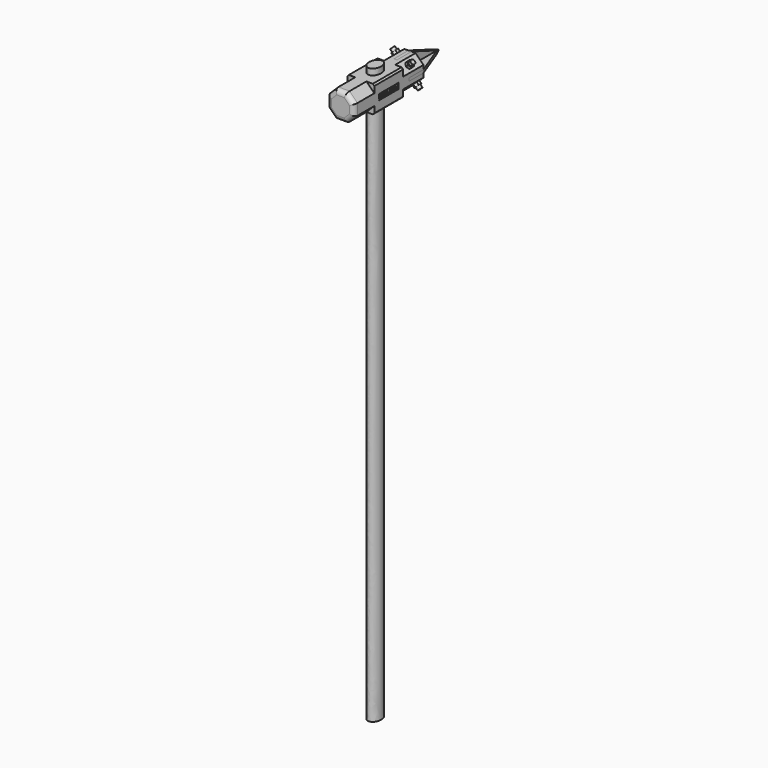
from build123d import *

# Parameters (mm, degrees)
F1_DEPTH       = 1219.2
F3_DEPTH       = 38.1
F3_DEPTH_BACK  = 38.1
F4_DEPTH       = 92.075
F4_DEPTH_BACK  = 92.075
F5_R           = 9.525
F6_SIZE        = 3.175
F7_DEPTH       = 1219.2
F8_W           = 51.7479172142
F8_H           = 12.878934881
F8_W_2         = 48.5729172142
F8_H_2         = 9.703934881
F8_TEXT_SIZE   = 9.0679651125
F9_DEPTH       = 0.79375
F10_W          = 51.7478878901
F10_H          = 12.8789306638
F10_W_2        = 48.5728878901
F10_H_2        = 9.7039306638
F10_TEXT_SIZE  = 9.0679592552
F11_DEPTH      = 0.79375
F13_DEPTH      = 38.1
F14_DEPTH      = 38.1
F15_DEPTH      = 76.2
F17_DEPTH      = 31.75
F17_DEPTH_BACK = 25.4
F19_DEPTH      = 25.4
F20_R          = 4.7625
F21_DEPTH      = 12.7
F21_DEPTH_BACK = 69.85
F22_DEPTH      = 6.35
F23_R          = 4.7625
F24_DEPTH      = 12.7
F24_DEPTH_BACK = 69.85
F25_DEPTH      = 6.35
F26_START      = -63.5
F22_FACE_R     = 4.7625
F26_DEPTH      = 6.35
F27_START      = -63.5
F25_FACE_R     = 4.7625
F27_DEPTH      = 6.35


# Not quite as in the source:
# - Text() gives the source's letters only with a copy of the font that has no kerning and outlines rounded to 1/6400 em; it was checked with that copy


with BuildPart() as f1:
    # F0 (on Top) → F1 (new body)
    with BuildSketch(Plane.XY):
        with BuildLine():
            add(Edge.make_bspline(
                [(12.7, 0), (12.7, 30.2459372272), (-6.35, 15.1229686136), (-25.4, 0), (-6.35, -15.1229686136), (12.7, -30.2459372272), (12.7, 0)],
                knots=[4.7123889804, 4.7123889804, 4.7123889804, 6.8067840828, 6.8067840828, 8.9011791852, 8.9011791852, 10.9955742876, 10.9955742876, 10.9955742876], degree=2, weights=[1, 0.5, 1, 0.5, 1, 0.5, 1]))
        make_face()
    extrude(amount=F1_DEPTH)


with BuildPart() as f3:
    # F2 (on Front) → F3 (new body, two sides)
    with BuildSketch(Plane.XZ) as f3_sk:
        Polygon((-28.575, 1189.7030929186), (-11.8361525448, 1206.4419403738), (-28.575, 1206.4419403738), align=None)
        Polygon((11.8361525448, 1206.4419403738), (28.575, 1189.7030929186), (28.575, 1206.4419403738), align=None)
        Polygon((28.575, 1166.030787829), (28.575, 1189.7030929186), (11.8361525448, 1206.4419403738), (-11.8361525448, 1206.4419403738), (-28.575, 1189.7030929186), (-28.575, 1166.030787829), (-11.8361525448, 1149.2919403738), (11.8361525448, 1149.2919403738), align=None)
        Polygon((-28.575, 1149.2919403738), (-11.8361525448, 1149.2919403738), (-28.575, 1166.030787829), align=None)
        Polygon((28.575, 1149.2919403738), (28.575, 1166.030787829), (11.8361525448, 1149.2919403738), align=None)
    extrude(amount=F3_DEPTH)
    extrude(f3_sk.sketch, amount=-F3_DEPTH_BACK)

    # F2 (on Front) → F4 (join, two sides)
    with BuildSketch(Plane.XZ) as f4_sk:
        Polygon((28.575, 1166.030787829), (28.575, 1189.7030929186), (11.8361525448, 1206.4419403738), (-11.8361525448, 1206.4419403738), (-28.575, 1189.7030929186), (-28.575, 1166.030787829), (-11.8361525448, 1149.2919403738), (11.8361525448, 1149.2919403738), align=None)
    extrude(amount=F4_DEPTH)
    extrude(f4_sk.sketch, amount=-F4_DEPTH_BACK)

    # F5
    f5_edges = [f3.edges().sort_by_distance(p)[0] for p in [
        (20.205576, -92.075, 1157.661364),
        (28.575, -92.075, 1177.86694),
        (20.205576, -92.075, 1198.072517),
        (0, -92.075, 1206.44194),
        (-20.205576, -92.075, 1198.072517),
        (-28.575, -92.075, 1177.86694),
        (-20.205576, -92.075, 1157.661364),
        (0, -92.075, 1149.29194),
    ]]
    fillet(f5_edges, radius=F5_R)

    # F6
    f6_edges = [f3.edges().sort_by_distance(p)[0] for p in [
        (28.575, 0, 1206.44194),
        (28.575, 0, 1149.29194),
        (-28.575, 0, 1206.44194),
        (-28.575, 0, 1149.29194),
    ]]
    chamfer(f6_edges, length=F6_SIZE)

    # F0 (on Top) → F7 (cut)
    with BuildSketch(Plane.XY):
        with BuildLine():
            add(Edge.make_bspline(
                [(12.7, 0), (12.7, 30.2459372272), (-6.35, 15.1229686136), (-25.4, 0), (-6.35, -15.1229686136), (12.7, -30.2459372272), (12.7, 0)],
                knots=[4.7123889804, 4.7123889804, 4.7123889804, 6.8067840828, 6.8067840828, 8.9011791852, 8.9011791852, 10.9955742876, 10.9955742876, 10.9955742876], degree=2, weights=[1, 0.5, 1, 0.5, 1, 0.5, 1]))
        make_face()
    extrude(amount=F7_DEPTH, mode=Mode.SUBTRACT)

    # F8 (on face) → F9 (cut)
    with BuildSketch(Plane.YZ.offset(28.575)):
        with Locations((0, 1177.8669403738)):
            Rectangle(F8_W, F8_H)
        with Locations((0, 1177.8669403738)):
            Rectangle(F8_W_2, F8_H_2, mode=Mode.SUBTRACT)
        with Locations((-22.6989586071, 1174.6024729333)):
            Text('ARTILLIER', F8_TEXT_SIZE, font='Open Sans', font_style=FontStyle.BOLD, text_align=(TextAlign.LEFT, TextAlign.BOTTOM))
    extrude(amount=-F9_DEPTH, mode=Mode.SUBTRACT)

    # F10 (on face) → F11 (cut)
    with BuildSketch(Plane(origin=(-28.575, 0, 0), x_dir=(0, -1, 0), z_dir=(-1, 0, 0))):
        with Locations((0, 1177.925)):
            Rectangle(F10_W, F10_H)
        with Locations((0, 1177.925)):
            Rectangle(F10_W_2, F10_H_2, mode=Mode.SUBTRACT)
        with Locations((-22.6989439451, 1174.6605346681)):
            Text('ARTILLIER', F10_TEXT_SIZE, font='Open Sans', font_style=FontStyle.BOLD, text_align=(TextAlign.LEFT, TextAlign.BOTTOM))
    extrude(amount=-F11_DEPTH, mode=Mode.SUBTRACT)

    # F12 (on face) → F13 (cut)
    with BuildSketch(Plane(origin=(0, 92.075, 0), x_dir=(-1, 0, 0), z_dir=(0, 1, 0))):
        Polygon((-3.175, 1149.2919403738), (3.175, 1149.2919403738), (3.175, 1174.6919403738), (28.575, 1174.6919403738), (28.575, 1181.0419403738), (3.175, 1181.0419403738), (3.175, 1206.4419403738), (-3.175, 1206.4419403738), (-3.175, 1181.0419403738), (-28.575, 1181.0419403738), (-28.575, 1174.6919403738), (-3.175, 1174.6919403738), align=None)
    extrude(amount=-F13_DEPTH, mode=Mode.SUBTRACT)


with BuildPart() as f14:
    # F12 (on face) → F14 (new body)
    with BuildSketch(Plane(origin=(0, 92.075, 0), x_dir=(-1, 0, 0), z_dir=(0, 1, 0))):
        Polygon((-3.175, 1149.2919403738), (3.175, 1149.2919403738), (3.175, 1174.6919403738), (28.575, 1174.6919403738), (28.575, 1181.0419403738), (3.175, 1181.0419403738), (3.175, 1206.4419403738), (-3.175, 1206.4419403738), (-3.175, 1181.0419403738), (-28.575, 1181.0419403738), (-28.575, 1174.6919403738), (-3.175, 1174.6919403738), align=None)
    extrude(amount=-F14_DEPTH)

    # F15 (add): a face of the model
    f15_faces = [f14.faces().sort_by_distance(p)[0] for p in [
        (0, 92.075, 1177.8669403738),
    ]]
    extrude(f15_faces, amount=F15_DEPTH)

    # F16 (on face) → F17 (cut, two sides)
    with BuildSketch(Plane.YZ.offset(3.175)) as f17_sk:
        Polygon((168.275, 1177.8669403738), (168.275, 1181.0419403738), (159.8083333333, 1181.0419403738), align=None)
        Polygon((168.275, 1149.2919403738), (168.275, 1177.8669403738), (92.075, 1149.2919403738), align=None)
        Polygon((168.275, 1181.0419403738), (168.275, 1206.4419403738), (92.075, 1206.4419403738), (159.8083333333, 1181.0419403738), align=None)
    extrude(amount=-F17_DEPTH, mode=Mode.SUBTRACT)
    extrude(f17_sk.sketch, amount=F17_DEPTH_BACK, mode=Mode.SUBTRACT)

    # F18 (on face) → F19 (cut)
    with BuildSketch(Plane.XY.offset(1181.0419403738)):
        Polygon((28.575, 92.075), (28.575, 159.8083333333), (3.175, 159.8083333333), align=None)
        Polygon((-28.575, 92.075), (0, 168.275), (-28.575, 168.275), align=None)
        Polygon((28.575, 159.8083333333), (28.575, 168.275), (0, 168.275), (3.175, 159.8083333333), align=None)
    extrude(amount=-F19_DEPTH, mode=Mode.SUBTRACT)

    # F20 (on face) → F21 (join, two sides)
    with BuildSketch(Plane(origin=(-609.1390464593, 0, 609.1390464593), x_dir=(0, -1, 0), z_dir=(-0.7071067812, 0, 0.7071067812))) as f21_sk:
        with Locations((-82.55, 832.8777008738)):
            Circle(F20_R)
    extrude(amount=F21_DEPTH)
    extrude(f21_sk.sketch, amount=-F21_DEPTH_BACK)

    # F20 (on face) → F22 (join)
    with BuildSketch(Plane(origin=(-609.1390464593, 0, 609.1390464593), x_dir=(0, -1, 0), z_dir=(-0.7071067812, 0, 0.7071067812))):
        Polygon((-86.121875, 826.6910318955), (-78.978125, 826.6910318955), (-75.40625, 832.8777008738), (-78.978125, 839.0643698521), (-86.121875, 839.0643698521), (-89.69375, 832.8777008738), align=None)
        with Locations((-82.55, 832.8777008738)):
            Circle(F20_R, mode=Mode.SUBTRACT)
    extrude(amount=F22_DEPTH)

    # F23 (on face) → F24 (join, two sides)
    with BuildSketch(Plane(origin=(609.1390464593, 0, 609.1390464593), x_dir=(0.7071067812, 0, -0.7071067812), z_dir=(0.7071067812, 0, 0.7071067812))) as f24_sk:
        with Locations((-832.8777008738, 63.5)):
            Circle(F23_R)
    extrude(amount=F24_DEPTH)
    extrude(f24_sk.sketch, amount=-F24_DEPTH_BACK)

    # F23 (on face) → F25 (join)
    with BuildSketch(Plane(origin=(609.1390464593, 0, 609.1390464593), x_dir=(0.7071067812, 0, -0.7071067812), z_dir=(0.7071067812, 0, 0.7071067812))):
        Polygon((-826.6910318955, 59.928125), (-826.6910318955, 67.071875), (-832.8777008738, 70.64375), (-839.0643698521, 67.071875), (-839.0643698521, 59.928125), (-832.8777008738, 56.35625), align=None)
        with Locations((-832.8777008738, 63.5)):
            Circle(F23_R, mode=Mode.SUBTRACT)
    extrude(amount=F25_DEPTH)

    # F22_face (on face) → F26 (join)
    with BuildSketch(Plane(origin=(-24.6957043329, 82.55, 1202.5626447068), x_dir=(0, -1, 0), z_dir=(-0.7071067812, 0, 0.7071067812)).offset(F26_START)):
        Polygon((-3.571875, -6.1866689783), (3.571875, -6.1866689783), (7.14375, 0), (3.571875, 6.1866689783), (-3.571875, 6.1866689783), (-7.14375, 0), align=None)
        Circle(F22_FACE_R, mode=Mode.SUBTRACT)
    extrude(amount=-F26_DEPTH)

    # F25_face (on face) → F27 (join)
    with BuildSketch(Plane(origin=(24.6957043329, 63.5, 1202.5626447068), x_dir=(0.7071067812, 0, -0.7071067812), z_dir=(0.7071067812, 0, 0.7071067812)).offset(F27_START)):
        Polygon((6.1866689783, -3.571875), (6.1866689783, 3.571875), (0, 7.14375), (-6.1866689783, 3.571875), (-6.1866689783, -3.571875), (0, -7.14375), align=None)
        Circle(F25_FACE_R, mode=Mode.SUBTRACT)
    extrude(amount=-F27_DEPTH)


solid = Compound([f1.part, f3.part, f14.part])
